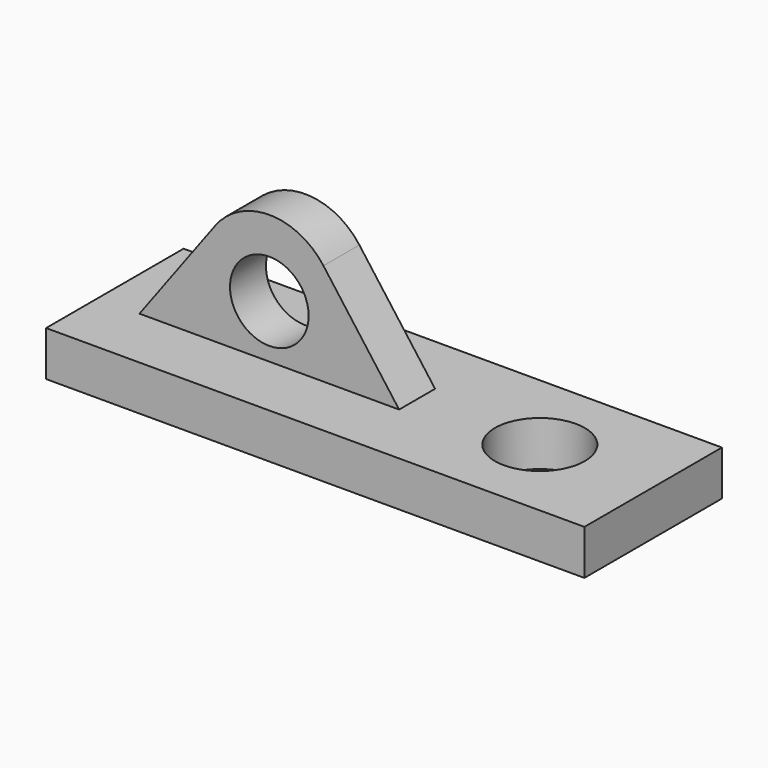
from build123d import *

# Parameters (mm, degrees)
F0_W     = 23.9590460792
F0_H     = 7.6507304548
F0_R     = 2
F1_DEPTH = 2
F2_R     = 1.75
F3_DEPTH = 1


# Not quite as in the source:
# - a feature names something its author has since deleted; it is built from what else it names


with BuildPart() as f1:
    # F0 (on Top) → F1 (new body)
    with BuildSketch(Plane.XY):
        with Locations((4.3424949229, -0.0471555286)):
            Rectangle(F0_W, F0_H)
        with Locations((11.2411081956, 0)):
            Circle(F0_R, mode=Mode.SUBTRACT)
    extrude(amount=F1_DEPTH)

    # F2 (on Front) → F3 (join, symmetric)
    with BuildSketch(Plane.XZ):
        with BuildLine():
            Line((-2.4094440999, 6.5410234491), (-5.7779996579, 2))
            Line((-5.7779996579, 2), (5.7779996579, 2))
            Line((5.7779996579, 2), (2.4094440999, 6.5410234491))
            ThreePointArc((2.4094440999, 6.5410234491), (0, 7.7536848887), (-2.4094440999, 6.5410234491))
        make_face()
        with Locations((0, 4.3635135517)):
            Circle(F2_R, mode=Mode.SUBTRACT)
    extrude(amount=F3_DEPTH, both=True)


solid = f1.part
